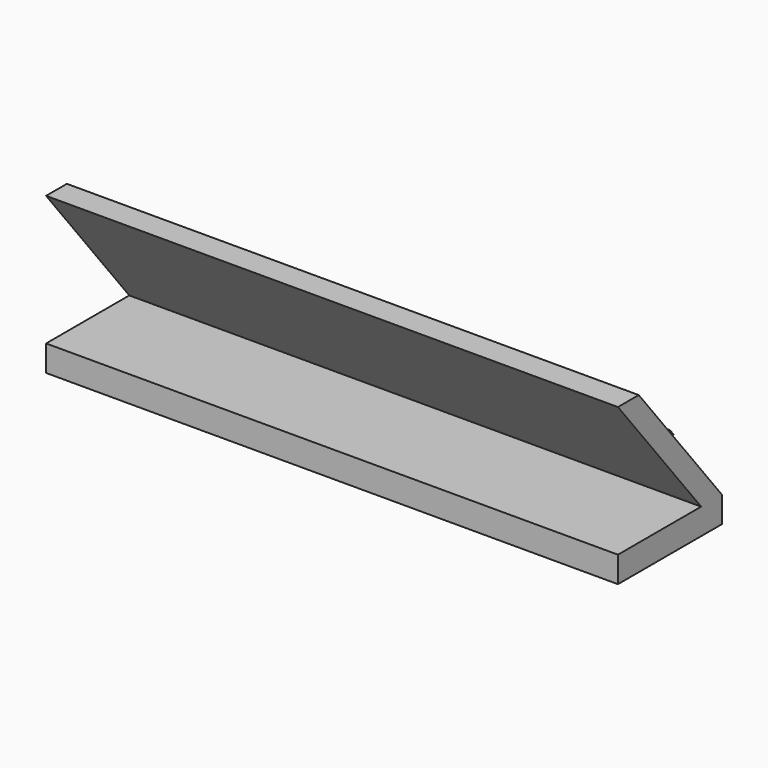
from build123d import *

# Parameters (mm, degrees)
F0_W           = 110
F0_H           = 30
F1_DEPTH       = 25
F3_DEPTH       = 115
F5_TEXT_SIZE   = 11.3680577876
F5_TEXT_SIZE_2 = 7.9875432361
F6_DEPTH       = 1


# Not quite as in the source:
# - Text() gives the source's letters only with a copy of the font that has no kerning and outlines rounded to 1/6400 em; it was checked with that copy


with BuildPart() as f1:
    # F0 (on Front) → F1 (new body)
    with BuildSketch(Plane.XZ):
        with Locations((5.9985700063, -15.1491501091)):
            Rectangle(F0_W, F0_H)
    extrude(amount=F1_DEPTH)

    # F2 (on face) → F3 (cut)
    with BuildSketch(Plane.YZ.offset(60.9985700063)):
        Polygon((-5, -25.1491501091), (-25, -0.1491501091), (-25, -25.1491501091), align=None)
        Polygon((-20, -0.1491501091), (0, -25.1491501091), (0, -0.1491501091), align=None)
    extrude(amount=-F3_DEPTH, mode=Mode.SUBTRACT)

    # F5 (on face) → F6 (join)
    with BuildSketch(Plane(origin=(0, -12.267878102, -9.8143024816), x_dir=(-1, 0, 0), z_dir=(0, 0.7808688094, 0.6246950476))):
        with Locations((-58.4985700063, -0.8075673241)):
            Text('Joshua Williamson', F5_TEXT_SIZE, font='Open Sans', font_style=FontStyle.BOLD, text_align=(TextAlign.LEFT, TextAlign.BOTTOM))
        with Locations((-58.4985700063, -14.6381869042)):
            Text('Professional GNU Emacs User', F5_TEXT_SIZE_2, font='Open Sans', font_style=FontStyle.ITALIC, text_align=(TextAlign.LEFT, TextAlign.BOTTOM))
    extrude(amount=F6_DEPTH)


solid = f1.part
